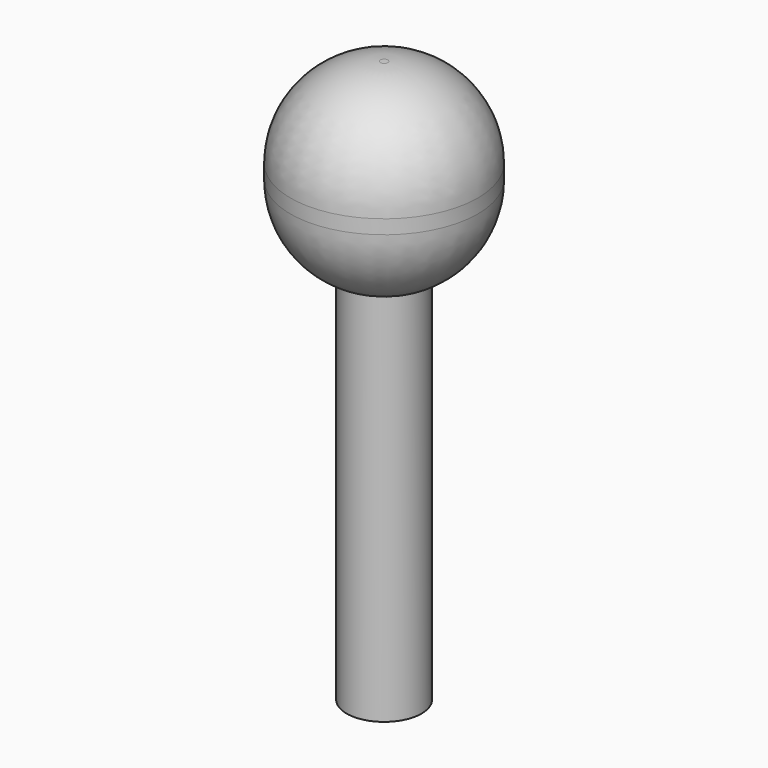
from build123d import *

# Parameters (mm, degrees)
F0_R     = 0.5
F1_DEPTH = 5
F2_R     = 1.25
F3_DEPTH = 2.5


# Not quite as in the source:
# - a fillet or chamfer that OpenCascade refuses, or shapes differently, is made with other operations: its cross-section is extruded or revolved along the edge and cut away or added


with BuildPart() as f1:
    # F0 (on Top) → F1 (new body)
    with BuildSketch(Plane.XY):
        Circle(F0_R)
    extrude(amount=F1_DEPTH)

    # F2 (on face) → F3 (join)
    with BuildSketch(Plane.XY.offset(5)):
        Circle(F2_R)
    extrude(amount=F3_DEPTH)

    # F4: fillet of radius 1.2 on 2 edges, made by hand

    # F4_s1 → F4_t2 (revolve, cut)
    with BuildSketch(Plane.XZ):
        with BuildLine():
            ThreePointArc((1.25, 6.3), (0.8985281374, 7.1485281374), (0.05, 7.5))
            Line((0.05, 7.5), (1.25, 7.5))
            Line((1.25, 7.5), (1.25, 6.3))
        make_face()
    revolve(axis=Axis((0, 0, 7.5), (0, 0, 1)), mode=Mode.SUBTRACT)

    # F4_s3 → F4_t4 (revolve, cut)
    with BuildSketch(Plane.XZ):
        with BuildLine():
            ThreePointArc((1.25, 6.1124297731), (1.0449874371, 5.4416093798), (0.5, 5))
            Line((0.5, 5), (1.25, 5))
            Line((1.25, 5), (1.25, 6.1124297731))
        make_face()
    revolve(axis=Axis((0, 0, 5), (0, 0, 1)), mode=Mode.SUBTRACT)


solid = f1.part
